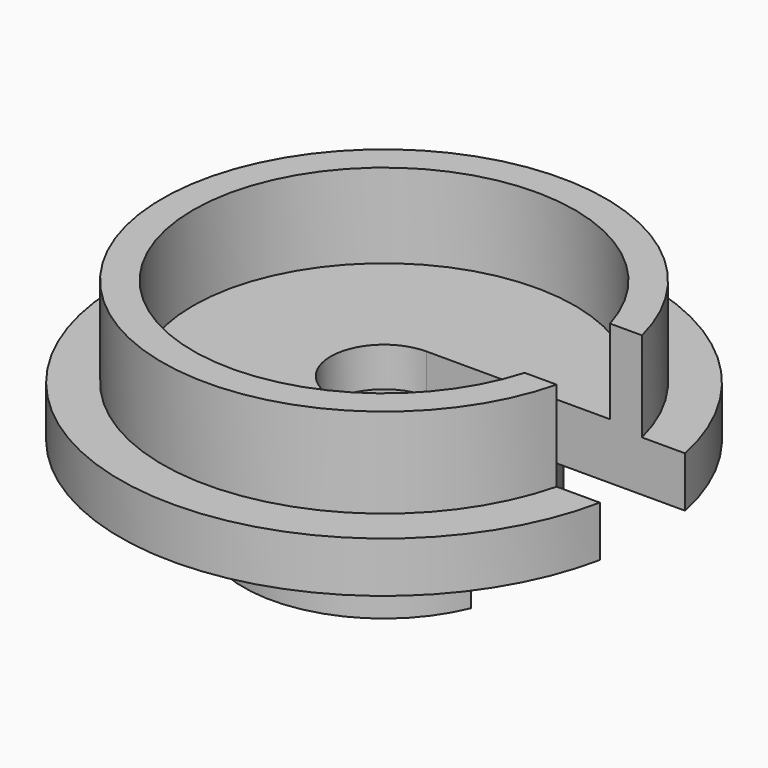
from build123d import *

# Parameters (mm, degrees)
F3_DEPTH      = 21
F3_DEPTH_BACK = 5.081


# Not quite as in the source:
# - an extrude ends at something that could not be found from the text; its depth is read off the source's solid


with BuildPart() as f1:
    # F0 (on Front) → F1 (revolve)
    with BuildSketch(Plane.XZ):
        Polygon((1.9685, 2.286), (1.9685, 0), (3.175, 0), (3.175, 1.905), (5.969, 1.905), (5.969, 3.048), (5.0165, 3.048), (5.0165, 5.08), (4.318, 5.08), (4.318, 3.175), (1.2065, 3.175), (1.2065, 2.286), align=None)
    revolve(axis=Axis((0, 0, 1.6013546669), (0, 0, -1)))

    # F2 (on Top) → F3 (cut, two sides)
    with BuildSketch(Plane.XY) as f3_sk:
        with BuildLine():
            Line((5.845794963, 1.2065), (0, 1.2065))
            ThreePointArc((0, 1.2065), (-1.2065, 0), (0, -1.2065))
            Line((0, -1.2065), (5.845794963, -1.2065))
            ThreePointArc((5.845794963, -1.2065), (5.969, 0), (5.845794963, 1.2065))
        make_face()
    extrude(amount=-F3_DEPTH, mode=Mode.SUBTRACT)
    extrude(f3_sk.sketch, amount=F3_DEPTH_BACK, mode=Mode.SUBTRACT)


solid = f1.part
